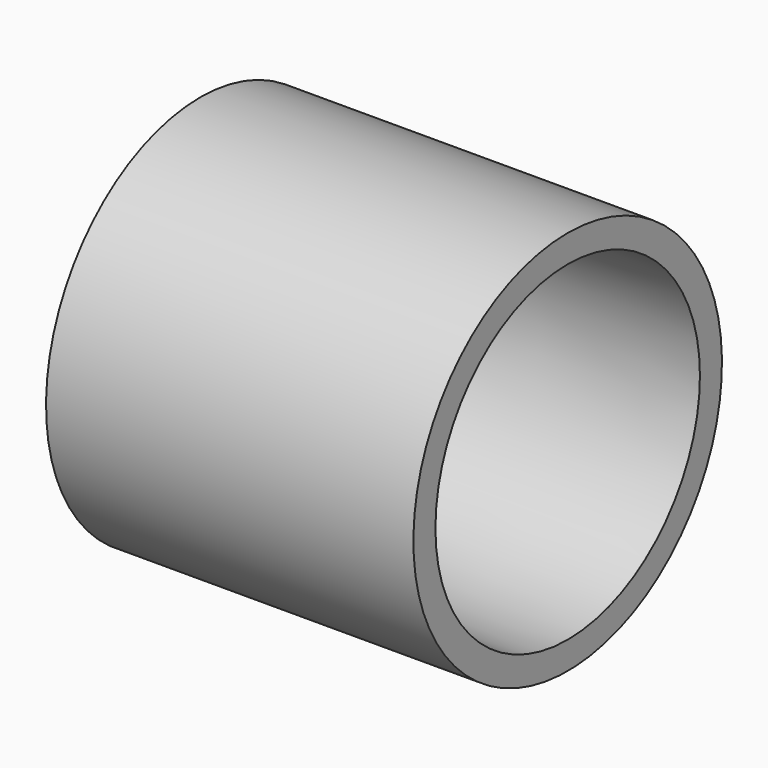
from build123d import *


# Not quite as in the source:
# - a feature of the source that left no trace in its solid (it failed there, or was rolled back) is left out


with BuildPart() as f1:
    # F0 (on Front) → F1 (revolve)
    with BuildSketch(Plane.XZ):
        Polygon((50.8, 26.67), (0, 26.67), (0, 22.098), (50.8, 22.86), align=None)
    revolve(axis=Axis((-51.9470935156, 0, 0), (-1, 0, 0)))


solid = f1.part
